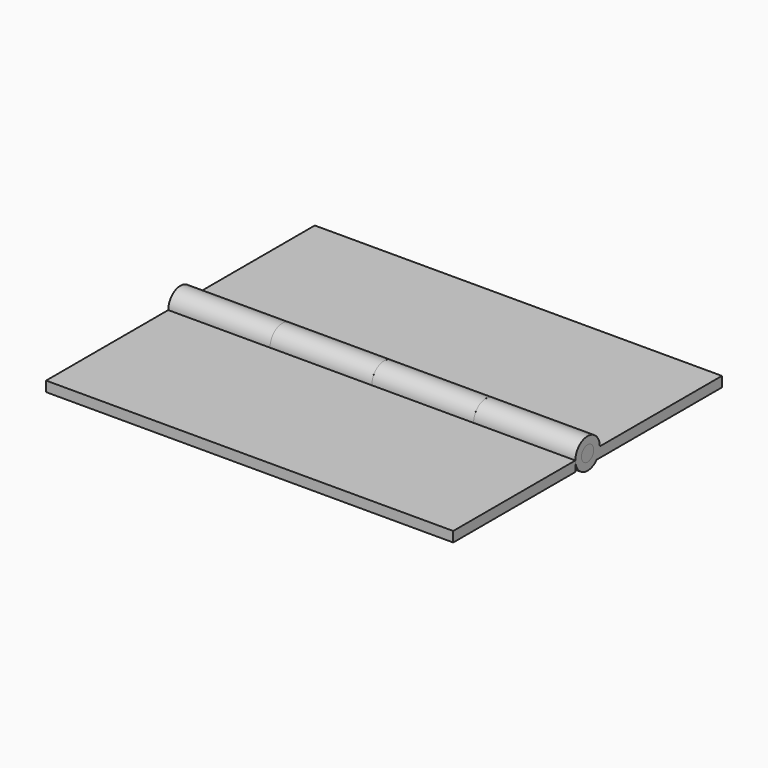
from build123d import *

# Parameters (mm, degrees)
F1_DEPTH = 2
F2_DEPTH = 2
F0_W     = 20
F0_H     = 3
F7_D     = 3
F7_2_D   = 3
F6_R     = 1.5
F8_DEPTH = 80


with BuildPart() as f1:
    # F0 (on Top) → F1 (new body)
    with BuildSketch(Plane.XY):
        Polygon((20, 15.0000010577), (40, 15.0000010577), (40, 48.0000031732), (-40, 48.0000031732), (-40, 18.0000010577), (-20, 18.0000010577), (-20, 15.0000010577), (0, 15.0000010577), (0, 18.0000010577), (20, 18.0000010577), align=None)
    extrude(amount=-F1_DEPTH)

    # F0 (on Top) → F4 (revolve)
    with BuildSketch(Plane.XY):
        with Locations((-10, 13.5000010577)):
            Rectangle(F0_W, F0_H)
        with Locations((30, 13.5000010577)):
            Rectangle(F0_W, F0_H)
    revolve(axis=Axis((0, 15.0000010577, 0), (1, 0, 0)))

    # F5: union 

    # F7 (through all)
    with Locations(Plane.YZ.offset(40)):
        with Locations((15.0000010577, 0)):
            Hole(F7_D / 2)


with BuildPart() as f2:
    # F0 (on Top) → F2 (new body)
    with BuildSketch(Plane.XY):
        Polygon((-40, -17.9999989423), (40, -18.0000010577), (40, 12.0000010577), (20, 12.0000010577), (20, 15.0000010577), (0, 15.0000010577), (0, 12.0000010577), (-20, 12.0000010577), (-20, 15.0000010577), (-40, 15.0000010577), align=None)
    extrude(amount=-F2_DEPTH)

    # F0 (on Top) → F3 (revolve)
    with BuildSketch(Plane.XY):
        with Locations((-30, 16.5000010577)):
            Rectangle(F0_W, F0_H)
        with Locations((10, 16.5000010577)):
            Rectangle(F0_W, F0_H)
    revolve(axis=Axis((0, 15.0000010577, 0), (1, 0, 0)))

    # F7#2 (through all)
    with Locations(Plane.YZ.offset(40)):
        with Locations((15.0000010577, 0)):
            Hole(F7_2_D / 2)


with BuildPart() as f8:
    # F6 (on face) → F8 (new body)
    with BuildSketch(Plane.YZ.offset(40)):
        with Locations((15.0000010577, 0)):
            Circle(F6_R)
    extrude(amount=-F8_DEPTH)


solid = Compound([f1.part, f2.part, f8.part])
